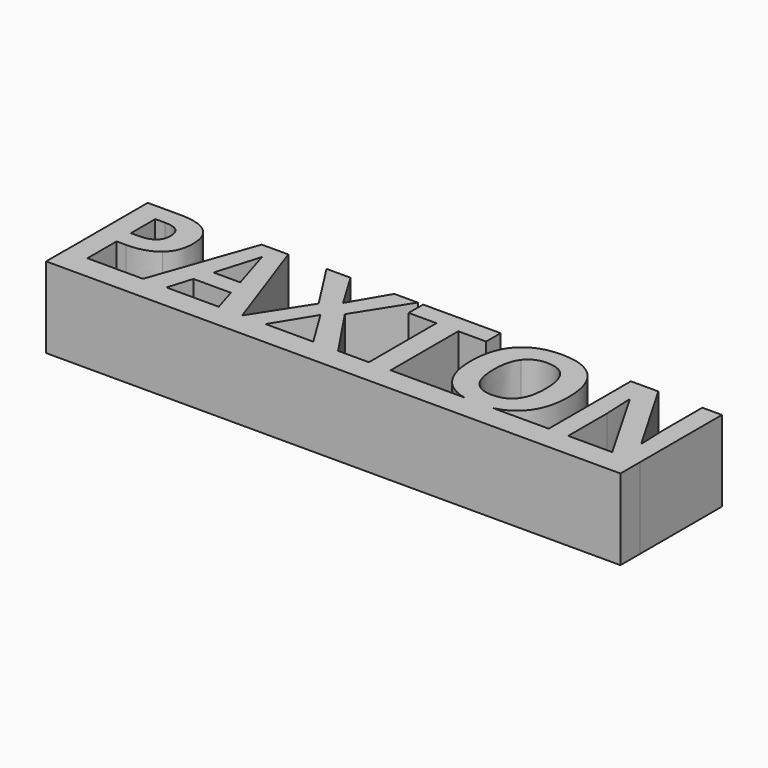
from build123d import *

# Parameters (mm, degrees)
F1_DEPTH = 12.7


# Not quite as in the source:
# - ends of sketch curves that miss each other by under 0.0002 mm in the source are joined


with BuildPart() as f1:
    # F0 (on Top) → F1 (new body)
    with BuildSketch(Plane.XY):
        with BuildLine():
            Line((261.5330806499, -47.4650785327), (261.5124285221, -47.4650785327))
            Line((261.5124285221, -47.4650785327), (261.5124285221, -51.2807406485))
            Line((261.5124285221, -51.2807406485), (351.8417477608, -51.2688159943))
            Line((351.8417477608, -51.2688159943), (351.8417477608, -47.4650785327))
            Line((351.8417477608, -47.4650785327), (347.4919441154, -47.4650785327))
            Line((347.4919441154, -47.4650785327), (340.5801815182, -47.4650785327))
            Line((340.5801815182, -47.4650785327), (337.5200657671, -47.4650785327))
            Line((337.5200657671, -47.4650785327), (328.6957807677, -47.4650785327))
            add(Edge.make_bspline(
                [(328.6957807677, -47.4650785327), (327.6809699352, -47.6876966532), (326.488101131, -47.6876966532)],
                knots=[0.6784981919, 0.6784981919, 0.6784981919, 1, 1, 1], degree=2))
            add(Edge.make_bspline(
                [(326.488101131, -47.6876966532), (325.2952323268, -47.6876966532), (324.2804214942, -47.4650785327)],
                knots=[0, 0, 0, 0.3215018081, 0.3215018081, 0.3215018081], degree=2))
            Line((324.2804214942, -47.4650785327), (312.6539750738, -47.4650785327))
            Line((312.6539750738, -47.4650785327), (309.2298963638, -47.4650785327))
            Line((309.2298963638, -47.4650785327), (304.39236927, -47.4650785327))
            Line((304.39236927, -47.4650785327), (300.4841844886, -47.4650785327))
            Line((300.4841844886, -47.4650785327), (292.9752399493, -47.4650785327))
            Line((292.9752399493, -47.4650785327), (289.3073413931, -47.4650785327))
            Line((289.3073413931, -47.4650785327), (285.6182411112, -47.4650785327))
            Line((285.6182411112, -47.4650785327), (277.391971517, -47.4650785327))
            Line((277.391971517, -47.4650785327), (273.7028712351, -47.4650785327))
            Line((273.7028712351, -47.4650785327), (264.9571593599, -47.4650785327))
            Line((264.9571593599, -47.4650785327), (261.5330806499, -47.4650785327))
        make_face()
        with BuildLine():
            Line((261.5330806499, -31.3199643679), (261.5330806499, -47.4650785327))
            Line((261.5330806499, -47.4650785327), (264.9571593599, -47.4650785327))
            Line((264.9571593599, -47.4650785327), (264.9571593599, -41.7229444732))
            Line((264.9571593599, -41.7229444732), (266.4236120581, -41.7229444732))
            add(Edge.make_bspline(
                [(271.0561891363, -40.3430654884), (269.4271898739, -41.7229444732), (266.4236120581, -41.7229444732)],
                knots=[0, 0, 0, 1, 1, 1], degree=2))
            add(Edge.make_bspline(
                [(272.6851883987, -36.3553742354), (272.6851883987, -38.9631865037), (271.0561891363, -40.3430654884)],
                knots=[0, 0, 0, 1, 1, 1], degree=2))
            add(Edge.make_bspline(
                [(271.1568973336, -32.5850006714), (272.6851883987, -33.850036975), (272.6851883987, -36.3553742354)],
                knots=[0, 0, 0, 1, 1, 1], degree=2))
            add(Edge.make_bspline(
                [(266.6886336301, -31.3199643679), (269.6286062686, -31.3199643679), (271.1568973336, -32.5850006714)],
                knots=[0, 0, 0, 1, 1, 1], degree=2))
            Line((266.6886336301, -31.3199643679), (261.5330806499, -31.3199643679))
        make_face()
        with BuildLine():
            Line((266.084384446, -38.9172494312), (264.9571593599, -38.9172494312))
            Line((264.9571593599, -38.9172494312), (264.9571593599, -34.1256594099))
            Line((264.9571593599, -34.1256594099), (266.5119525821, -34.1256594099))
            add(Edge.make_bspline(
                [(268.5720536016, -34.6998728158), (267.9148001031, -34.1256594099), (266.5119525821, -34.1256594099)],
                knots=[0, 0, 0, 1, 1, 1], degree=2))
            add(Edge.make_bspline(
                [(269.2293071001, -36.479050969), (269.2293071001, -35.2740862218), (268.5720536016, -34.6998728158)],
                knots=[0, 0, 0, 1, 1, 1], degree=2))
            add(Edge.make_bspline(
                [(268.4448432471, -38.2935653318), (269.2293071001, -37.6698812324), (269.2293071001, -36.479050969)],
                knots=[0, 0, 0, 1, 1, 1], degree=2))
            add(Edge.make_bspline(
                [(266.084384446, -38.9172494312), (267.660379394, -38.9172494312), (268.4448432471, -38.2935653318)],
                knots=[0, 0, 0, 1, 1, 1], degree=2))
        make_face(mode=Mode.SUBTRACT)
        with BuildLine():
            Line((347.4919441154, -47.4650785327), (351.8417477608, -47.4650785327))
            Line((351.8417477608, -47.4650785327), (351.8418315167, -31.3199643679))
            Line((351.8418315167, -31.3199643679), (348.7605140399, -31.3199643679))
            Line((348.7605140399, -31.3199643679), (348.7605140399, -38.9631865037))
            add(Edge.make_bspline(
                [(348.926594225, -43.4120152919), (348.7605140399, -40.2635590168), (348.7605140399, -38.9631865037)],
                knots=[0, 0, 0, 1, 1, 1], degree=2))
            Line((348.926594225, -43.4120152919), (348.8488545639, -43.4120152919))
            Line((348.8488545639, -43.4120152919), (341.8381505799, -31.3199643679))
            Line((341.8381505799, -31.3199643679), (337.5200657671, -31.3199643679))
            Line((337.5200657671, -31.3199643679), (337.5200657671, -47.4650785327))
            Line((337.5200657671, -47.4650785327), (340.5801815182, -47.4650785327))
            Line((340.5801815182, -47.4650785327), (340.5801815182, -39.8677934694))
            add(Edge.make_bspline(
                [(340.3681642606, -35.252884496), (340.5801815182, -38.4861476741), (340.5801815182, -39.8677934694)],
                knots=[0, 0, 0, 1, 1, 1], degree=2))
            Line((340.3681642606, -35.252884496), (340.4671056475, -35.252884496))
            Line((340.4671056475, -35.252884496), (347.4919441154, -47.4650785327))
        make_face()
        Polygon((279.4026018431, -31.2528255696), (273.7028712351, -47.4650785327), (277.391971517, -47.4650785327), (278.5616000547, -43.6204989286), (284.4486125735, -43.6204989286), (285.6182411112, -47.4650785327), (289.3073413931, -47.4650785327), (283.5864090594, -31.2528255696), align=None)
        with BuildLine():
            add(Edge.make_bspline(
                [(283.6288125109, -40.7511987093), (282.0068804904, -35.5285069309), (281.8019304747, -34.8429844647)],
                knots=[0, 0, 0, 1, 1, 1], degree=2))
            Line((283.6288125109, -40.7511987093), (279.4238035688, -40.7511987093))
            add(Edge.make_bspline(
                [(281.5086399351, -33.761696451), (281.1446769762, -35.1751448349), (279.4238035688, -40.7511987093)],
                knots=[0, 0, 0, 1, 1, 1], degree=2))
            add(Edge.make_bspline(
                [(281.8019304747, -34.8429844647), (281.596980459, -34.1574619985), (281.5086399351, -33.761696451)],
                knots=[0, 0, 0, 1, 1, 1], degree=2))
        make_face(mode=Mode.SUBTRACT)
        Polygon((294.664310768, -39.1398675517), (289.3073413931, -47.4650785327), (292.9752399493, -47.4650785327), (296.7279454084, -41.3589815143), (300.4841844886, -47.4650785327), (304.39236927, -47.4650785327), (298.9364585083, -39.3271494625), (304.0036709644, -31.3199643679), (300.3181043035, -31.3199643679), (296.9046264564, -37.1292372256), (293.4275434321, -31.3199643679), (289.6501026262, -31.3199643679), align=None)
        with BuildLine():
            add(Edge.make_bspline(
                [(328.6957807677, -47.4650785327), (327.6809699352, -47.6876966532), (326.488101131, -47.6876966532)],
                knots=[0.6784981919, 0.6784981919, 0.6784981919, 1, 1, 1], degree=2))
            Line((328.6957807677, -47.4650785327), (324.2804214942, -47.4650785327))
            add(Edge.make_bspline(
                [(326.488101131, -47.6876966532), (325.2952323268, -47.6876966532), (324.2804214942, -47.4650785327)],
                knots=[0, 0, 0, 0.3215018081, 0.3215018081, 0.3215018081], degree=2))
        make_face()
        with BuildLine():
            Line((324.2804214942, -47.4650785327), (328.6957807677, -47.4650785327))
            add(Edge.make_bspline(
                [(332.1860649285, -45.5339546782), (330.837439998, -46.995264714), (328.6957807677, -47.4650785327)],
                knots=[0, 0, 0, 0.6784981919, 0.6784981919, 0.6784981919], degree=2))
            add(Edge.make_bspline(
                [(334.1737267183, -39.369552914), (334.1737267183, -43.3802127033), (332.1860649285, -45.5339546782)],
                knots=[0, 0, 0, 1, 1, 1], degree=2))
            add(Edge.make_bspline(
                [(332.2019662228, -33.2086847708), (334.1737267183, -35.3518258829), (334.1737267183, -39.369552914)],
                knots=[0, 0, 0, 1, 1, 1], degree=2))
            add(Edge.make_bspline(
                [(326.5093028567, -31.0655436588), (330.2302057273, -31.0655436588), (332.2019662228, -33.2086847708)],
                knots=[0, 0, 0, 1, 1, 1], degree=2))
            add(Edge.make_bspline(
                [(320.7954377649, -33.191016666), (322.7883999862, -31.0655436588), (326.5093028567, -31.0655436588)],
                knots=[0, 0, 0, 1, 1, 1], degree=2))
            add(Edge.make_bspline(
                [(318.8024755436, -39.3483511883), (318.8024755436, -35.3164896733), (320.7954377649, -33.191016666)],
                knots=[0, 0, 0, 1, 1, 1], degree=2))
            add(Edge.make_bspline(
                [(320.7901373335, -45.5339546782), (318.8024755436, -43.3802127033), (318.8024755436, -39.3483511883)],
                knots=[0, 0, 0, 1, 1, 1], degree=2))
            add(Edge.make_bspline(
                [(324.2804214942, -47.4650785327), (322.1387622639, -46.995264714), (320.7901373335, -45.5339546782)],
                knots=[0.3215018081, 0.3215018081, 0.3215018081, 1, 1, 1], degree=2))
        make_face()
        with BuildLine():
            add(Edge.make_bspline(
                [(322.3926344387, -39.369552914), (322.3926344387, -42.0763065692), (323.4191513275, -43.445584691)],
                knots=[0, 0, 0, 1, 1, 1], degree=2))
            add(Edge.make_bspline(
                [(323.4297521903, -35.2917543266), (322.3926344387, -36.6663328799), (322.3926344387, -39.369552914)],
                knots=[0, 0, 0, 1, 1, 1], degree=2))
            add(Edge.make_bspline(
                [(326.5093028567, -33.9171757732), (324.466869942, -33.9171757732), (323.4297521903, -35.2917543266)],
                knots=[0, 0, 0, 1, 1, 1], degree=2))
            add(Edge.make_bspline(
                [(330.5835678232, -39.369552914), (330.5835678232, -33.9171757732), (326.5093028567, -33.9171757732)],
                knots=[0, 0, 0, 1, 1, 1], degree=2))
            add(Edge.make_bspline(
                [(326.488101131, -44.8148628129), (330.5835678232, -44.8148628129), (330.5835678232, -39.369552914)],
                knots=[0, 0, 0, 1, 1, 1], degree=2))
            add(Edge.make_bspline(
                [(323.4191513275, -43.445584691), (324.4456682163, -44.8148628129), (326.488101131, -44.8148628129)],
                knots=[0, 0, 0, 1, 1, 1], degree=2))
        make_face(mode=Mode.SUBTRACT)
        Polygon((309.2298963638, -47.4650785327), (312.6539750738, -47.4650785327), (312.6539750738, -34.1680628614), (317.0356650638, -34.1680628614), (317.0356650638, -31.3199643679), (304.8446727529, -31.3199643679), (304.8446727529, -34.1680628614), (309.2298963638, -34.1680628614), align=None)
    extrude(amount=F1_DEPTH)


solid = f1.part
